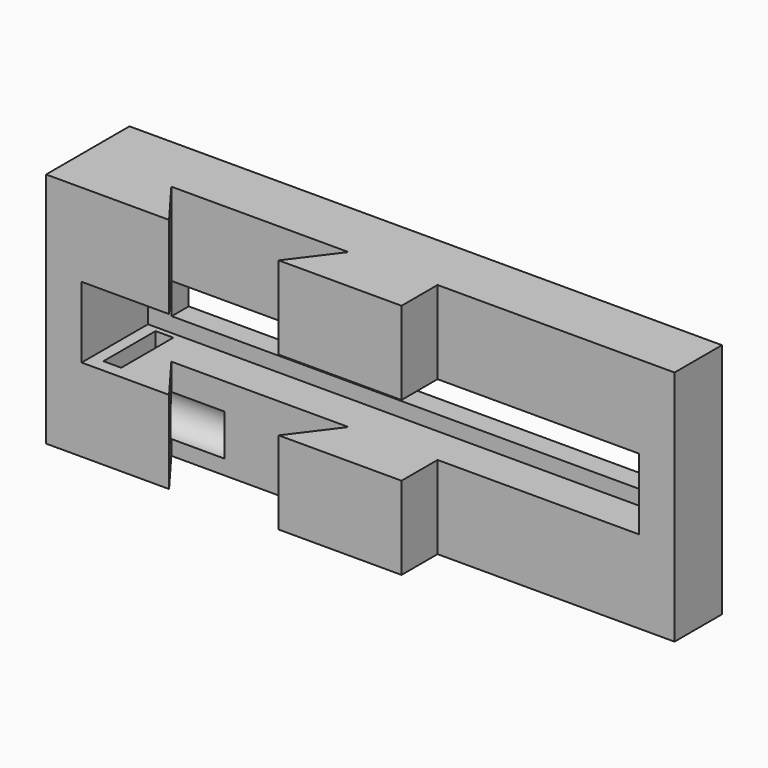
from build123d import *

# Parameters (mm, degrees)
F0_W      = 50
F0_H      = 20
F1_DEPTH  = 5
F2_W      = 30
F2_H      = 20
F3_DEPTH  = 3.8
F4_W      = 15.25
F4_H      = 20
F5_DEPTH  = 4
F6_SIZE2  = 3.99999
F6_SIZE   = 2.99999
F9_W      = 40
F9_H      = 3.5
F10_DEPTH = 12.5
F11_W     = 44
F11_H     = 6
F12_DEPTH = 7
F13_R     = 1.75
F14_DEPTH = 12
F15_W     = 1.5
F15_H     = 5.5
F16_DEPTH = 8


# Not quite as in the source:
# - a fillet or chamfer is up to 0.001 mm smaller than in the source, because OpenCascade refuses the exact size


with BuildPart() as f1:
    # F0 (on Front) → F1 (new body)
    with BuildSketch(Plane.XZ):
        Rectangle(F0_W, F0_H)
    extrude(amount=F1_DEPTH)


with BuildPart() as f3:
    # F2 (on face) → F3 (new body)
    with BuildSketch(Plane.XZ.offset(5)):
        with Locations((-10, 0)):
            Rectangle(F2_W, F2_H)
    extrude(amount=F3_DEPTH)


with BuildPart() as f5:
    # F4 (on face) → F5 (new body)
    with BuildSketch(Plane.XZ.offset(8.8)):
        with Locations((-9.995, 0)):
            Rectangle(F4_W, F4_H)
    extrude(amount=-F5_DEPTH)

    # F6 (size 3 and 4 in the source; OpenCascade refuses exactly that, so slightly less here)
    f6_edges = [f5.edges().sort_by_distance(p)[0] for p in [
        (-2.37, -8.8, 0),
        (-17.62, -8.8, 0),
    ]]
    f6_side = f5.faces().sort_by_distance((-9.995, -8.8, 0))[0]
    chamfer(f6_edges, length=F6_SIZE, length2=F6_SIZE2, reference=f6_side)


with BuildPart() as f3_1:
    add(f3.part)

    # F7: cut F5
    add(f5.part, mode=Mode.SUBTRACT)


with BuildPart() as f1_1:
    add(f1.part)

    # F8: union F3
    add(f3_1.part)

    # F9 (on face) → F10 (cut, symmetric)
    with BuildSketch(Plane.XZ.offset(8.8)):
        Rectangle(F9_W, F9_H)
    extrude(amount=F10_DEPTH, both=True, mode=Mode.SUBTRACT)

    # F11 (on face) → F12 (cut)
    with BuildSketch(Plane.XZ.offset(8.8)):
        Rectangle(F11_W, F11_H)
    extrude(amount=-F12_DEPTH, mode=Mode.SUBTRACT)

    # F13 (on face) → F14 (cut)
    with BuildSketch(Plane(origin=(-25, 0, 0), x_dir=(0, -1, 0), z_dir=(-1, 0, 0))):
        with Locations((5, -7)):
            Circle(F13_R)
    extrude(amount=-F14_DEPTH, mode=Mode.SUBTRACT)

    # F15 (on face) → F16 (cut)
    with BuildSketch(Plane(origin=(0, 0, -10), x_dir=(1, 0, 0), z_dir=(0, 0, -1))):
        with Locations((-20.25, 5)):
            Rectangle(F15_W, F15_H)
    extrude(amount=-F16_DEPTH, mode=Mode.SUBTRACT)


solid = f1_1.part
